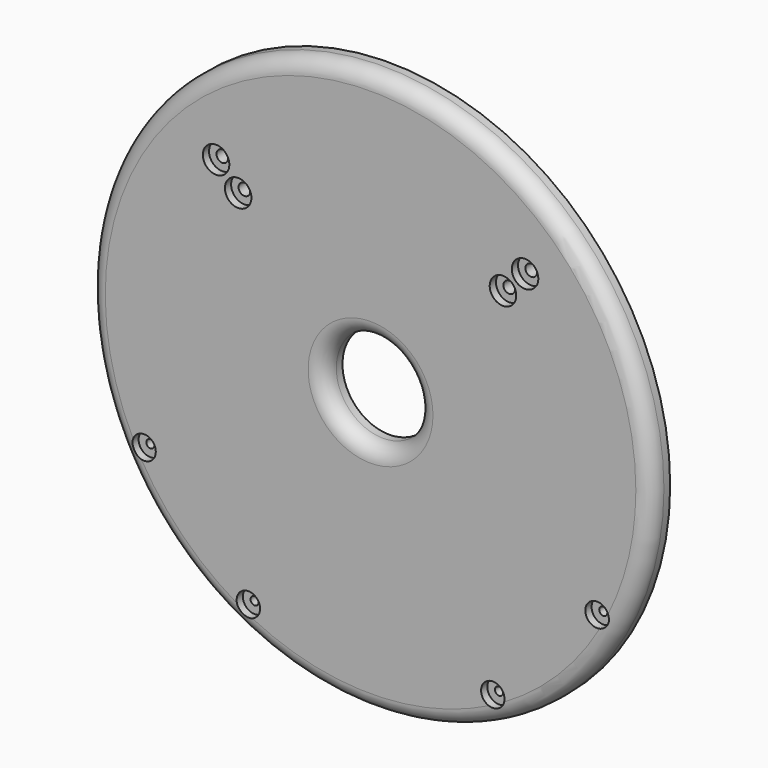
from build123d import *

# Parameters (mm, degrees)
F0_R     = 228.6
F1_DEPTH = 19.05
F2_R     = 38.1
F3_DEPTH = 19.051
F4_R     = 4.7625
F4_R_2   = 3.302
F5_DEPTH = 19.051
F6_R     = 10.795
F6_R_2   = 9.525
F7_DEPTH = 6.35


# Not quite as in the source:
# - a fillet or chamfer that OpenCascade refuses, or shapes differently, is made with other operations: its cross-section is extruded or revolved along the edge and cut away or added


with BuildPart() as f1:
    # F0 (on Front) → F1 (new body)
    with BuildSketch(Plane.XZ):
        Circle(F0_R)
    extrude(amount=F1_DEPTH)

    # F2 (on face) → F3 (cut, through all)
    with BuildSketch(Plane.XZ.offset(19.05)):
        Circle(F2_R)
    extrude(amount=-F3_DEPTH, mode=Mode.SUBTRACT)

    # F4 (on face) → F5 (cut, through all)
    with BuildSketch(Plane.XZ.offset(19.05)):
        with Locations((107.7630734528, 107.7630734528)):
            Circle(F4_R)
        with Locations((125.723585695, 125.723585695)):
            Circle(F4_R)
        with Locations((-107.7630734528, 107.7630734528)):
            Circle(F4_R)
        with Locations((-125.723585695, 125.723585695)):
            Circle(F4_R)
        with Locations((-99.4616398417, -184.3144535841)):
            Circle(F4_R_2)
        with Locations((-184.3144535841, -99.4616398417)):
            Circle(F4_R_2)
        with Locations((99.4616398417, -184.3144535841)):
            Circle(F4_R_2)
        with Locations((184.3144535841, -99.4616398417)):
            Circle(F4_R_2)
    extrude(amount=-F5_DEPTH, mode=Mode.SUBTRACT)

    # F6 (on face) → F7 (cut)
    with BuildSketch(Plane.XZ.offset(19.05)):
        with Locations((107.7630734528, 107.7630734528)):
            Circle(F6_R)
        with Locations((125.723585695, 125.723585695)):
            Circle(F6_R)
        with Locations((-125.723585695, 125.723585695)):
            Circle(F6_R)
        with Locations((-107.7630734528, 107.7630734528)):
            Circle(F6_R)
        with Locations((-184.3144535841, -99.4616398417)):
            Circle(F6_R_2)
        with Locations((-99.4616398417, -184.3144535841)):
            Circle(F6_R_2)
        with Locations((99.4616398417, -184.3144535841)):
            Circle(F6_R_2)
        with Locations((184.3144535841, -99.4616398417)):
            Circle(F6_R_2)
    extrude(amount=-F7_DEPTH, mode=Mode.SUBTRACT)

    # F8: fillet of radius 12.7 on 2 edges, made by hand

    # F8_s1 → F8_t2 (revolve, cut)
    with BuildSketch(Plane.XY):
        with BuildLine():
            ThreePointArc((228.6, -6.35), (224.8802561211, -15.3302561211), (215.9, -19.05))
            Line((215.9, -19.05), (228.6, -19.05))
            Line((228.6, -19.05), (228.6, -6.35))
        make_face()
    revolve(axis=Axis((0, -19.05, 0), (0, -1, 0)), mode=Mode.SUBTRACT)

    # F8_s3 → F8_t4 (revolve, cut)
    with BuildSketch(Plane.XY):
        with BuildLine():
            ThreePointArc((50.8, -19.05), (41.8197438789, -15.3302561211), (38.1, -6.35))
            Line((38.1, -6.35), (38.1, -19.05))
            Line((38.1, -19.05), (50.8, -19.05))
        make_face()
    revolve(axis=Axis((0, -19.05, 0), (0, -1, 0)), mode=Mode.SUBTRACT)


solid = f1.part
